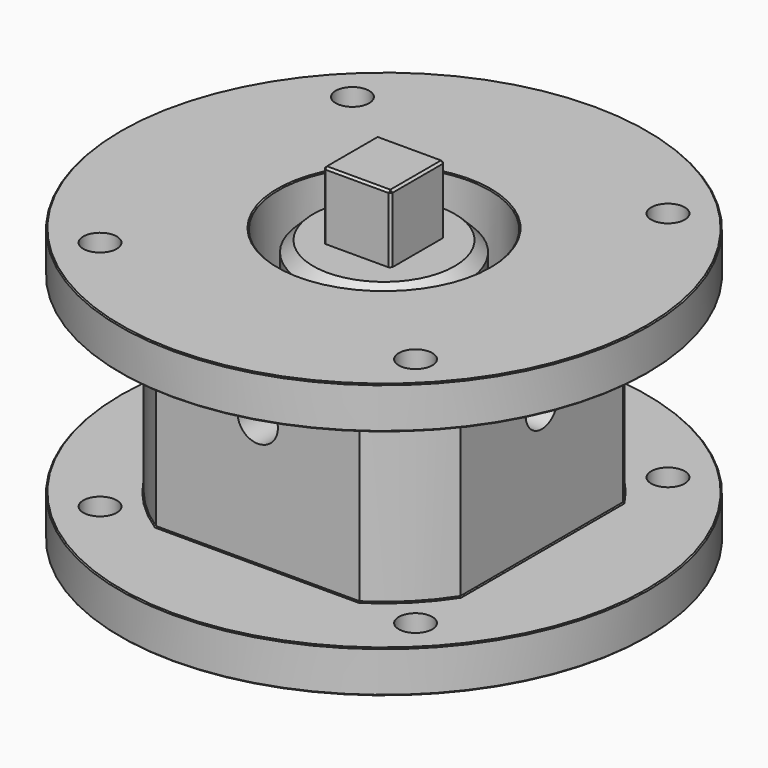
from build123d import *

# Parameters (mm, degrees)
F0_R      = 125
F0_R_2    = 50
F1_DEPTH  = 20
F2_DEPTH  = 45
F7_R      = 38.4930993585
F8_DEPTH  = 125
F9_W      = 32
F9_H      = 32
F10_DEPTH = 32
F11_W     = 32
F11_H     = 32
F12_DEPTH = 32
F13_SIZE  = 1
F14_SIZE  = 0.5
F15_D     = 15.875
F16_D     = 19.05
F16_2_D   = 19.05
F17_D     = 19.05
F17_DEPTH = 30
F17_TIP   = 5.7231973962
F19_D     = 19.05
F19_DEPTH = 30
F19_TIP   = 5.7231973962
F20_SIZE  = 5


# Not quite as in the source:
# - a length typed as a fraction of an inch, garbled in the dataset ("3 / 203.2 mm" for 3/8 in), is restored


with BuildPart() as f1:
    # F0 (on Top) → F1 (new body)
    with BuildSketch(Plane.XY):
        Circle(F0_R)
        with BuildLine():
            Line((-48.1726635133, -74.7033618391), (-74.7033618391, -74.7033618391))
            Line((-74.7033618391, -74.7033618391), (-74.7033618391, -48.1726635133))
            ThreePointArc((-74.7033618391, -48.1726635133), (-88.8886819568, 0), (-74.7033618391, 48.1726635133))
            Line((-74.7033618391, 48.1726635133), (-74.7033618391, 74.7033618391))
            Line((-74.7033618391, 74.7033618391), (-48.1726635133, 74.7033618391))
            ThreePointArc((-48.1726635133, 74.7033618391), (0, 88.8886819568), (48.1726635133, 74.7033618391))
            Line((48.1726635133, 74.7033618391), (74.7033618391, 74.7033618391))
            Line((74.7033618391, 74.7033618391), (74.7033618391, 48.1726635133))
            ThreePointArc((74.7033618391, 48.1726635133), (85.2686377036, 25.1089068699), (88.8886819568, 0))
            ThreePointArc((88.8886819568, 0), (85.2686377036, -25.1089068699), (74.7033618391, -48.1726635133))
            Line((74.7033618391, -48.1726635133), (74.7033618391, -74.7033618391))
            Line((74.7033618391, -74.7033618391), (48.1726635133, -74.7033618391))
            ThreePointArc((48.1726635133, -74.7033618391), (0, -88.8886819568), (-48.1726635133, -74.7033618391))
        make_face(mode=Mode.SUBTRACT)
        with BuildLine():
            Line((-74.7033618391, 48.1726635133), (-74.7033618391, -48.1726635133))
            ThreePointArc((-74.7033618391, -48.1726635133), (-62.8537897824, -62.8537897824), (-48.1726635133, -74.7033618391))
            Line((-48.1726635133, -74.7033618391), (48.1726635133, -74.7033618391))
            ThreePointArc((48.1726635133, -74.7033618391), (62.8537897824, -62.8537897824), (74.7033618391, -48.1726635133))
            Line((74.7033618391, -48.1726635133), (74.7033618391, 48.1726635133))
            ThreePointArc((74.7033618391, 48.1726635133), (62.8537897824, 62.8537897824), (48.1726635133, 74.7033618391))
            Line((48.1726635133, 74.7033618391), (-48.1726635133, 74.7033618391))
            ThreePointArc((-48.1726635133, 74.7033618391), (-62.8537897824, 62.8537897824), (-74.7033618391, 48.1726635133))
        make_face()
        Circle(F0_R_2, mode=Mode.SUBTRACT)
        with BuildLine():
            Line((48.1726635133, -74.7033618391), (-48.1726635133, -74.7033618391))
            ThreePointArc((-48.1726635133, -74.7033618391), (0, -88.8886819568), (48.1726635133, -74.7033618391))
        make_face()
        with BuildLine():
            ThreePointArc((-74.7033618391, 48.1726635133), (-88.8886819568, 0), (-74.7033618391, -48.1726635133))
            Line((-74.7033618391, -48.1726635133), (-74.7033618391, 48.1726635133))
        make_face()
        with BuildLine():
            ThreePointArc((48.1726635133, 74.7033618391), (0, 88.8886819568), (-48.1726635133, 74.7033618391))
            Line((-48.1726635133, 74.7033618391), (48.1726635133, 74.7033618391))
        make_face()
        with BuildLine():
            Line((74.7033618391, 48.1726635133), (74.7033618391, -48.1726635133))
            ThreePointArc((74.7033618391, -48.1726635133), (85.2686377036, -25.1089068699), (88.8886819568, 0))
            ThreePointArc((88.8886819568, 0), (85.2686377036, 25.1089068699), (74.7033618391, 48.1726635133))
        make_face()
        with BuildLine():
            Line((-74.7033618391, 74.7033618391), (-74.7033618391, 48.1726635133))
            ThreePointArc((-74.7033618391, 48.1726635133), (-62.8537897824, 62.8537897824), (-48.1726635133, 74.7033618391))
            Line((-48.1726635133, 74.7033618391), (-74.7033618391, 74.7033618391))
        make_face()
        with BuildLine():
            Line((-74.7033618391, -48.1726635133), (-74.7033618391, -74.7033618391))
            Line((-74.7033618391, -74.7033618391), (-48.1726635133, -74.7033618391))
            ThreePointArc((-48.1726635133, -74.7033618391), (-62.8537897824, -62.8537897824), (-74.7033618391, -48.1726635133))
        make_face()
        with BuildLine():
            ThreePointArc((74.7033618391, -48.1726635133), (62.8537897824, -62.8537897824), (48.1726635133, -74.7033618391))
            Line((48.1726635133, -74.7033618391), (74.7033618391, -74.7033618391))
            Line((74.7033618391, -74.7033618391), (74.7033618391, -48.1726635133))
        make_face()
        with BuildLine():
            Line((74.7033618391, 74.7033618391), (48.1726635133, 74.7033618391))
            ThreePointArc((48.1726635133, 74.7033618391), (62.8537897824, 62.8537897824), (74.7033618391, 48.1726635133))
            Line((74.7033618391, 48.1726635133), (74.7033618391, 74.7033618391))
        make_face()
    extrude(amount=-F1_DEPTH)

    # F0 (on Top) → F2 (join)
    with BuildSketch(Plane.XY):
        with BuildLine():
            Line((-74.7033618391, 48.1726635133), (-74.7033618391, -48.1726635133))
            ThreePointArc((-74.7033618391, -48.1726635133), (-62.8537897824, -62.8537897824), (-48.1726635133, -74.7033618391))
            Line((-48.1726635133, -74.7033618391), (48.1726635133, -74.7033618391))
            ThreePointArc((48.1726635133, -74.7033618391), (62.8537897824, -62.8537897824), (74.7033618391, -48.1726635133))
            Line((74.7033618391, -48.1726635133), (74.7033618391, 48.1726635133))
            ThreePointArc((74.7033618391, 48.1726635133), (62.8537897824, 62.8537897824), (48.1726635133, 74.7033618391))
            Line((48.1726635133, 74.7033618391), (-48.1726635133, 74.7033618391))
            ThreePointArc((-48.1726635133, 74.7033618391), (-62.8537897824, 62.8537897824), (-74.7033618391, 48.1726635133))
        make_face()
        Circle(F0_R_2, mode=Mode.SUBTRACT)
    extrude(amount=F2_DEPTH)

    # F3: F1 across face


with BuildPart() as f1_1:
    add(f1.part)
    add(f1.part.mirror(Plane.XY.offset(45)))

    # F14
    f14_edges = [f1_1.edges().sort_by_distance(p)[0] for p in [
        (-125, 0, 110),
        (-50, 0, 110),
        (-125, 0, 90),
        (-62.85379, 62.85379, 90),
        (-74.703362, 0, 90),
        (-62.85379, -62.85379, 90),
        (0, -74.703362, 90),
        (62.85379, -62.85379, 90),
        (74.703362, 0, 90),
        (62.85379, 62.85379, 90),
        (0, 74.703362, 90),
        (-125, 0, -20),
        (-50, 0, -20),
        (-125, 0, 0),
        (-62.85379, 62.85379, 0),
        (-74.703362, 0, 0),
        (-62.85379, -62.85379, 0),
        (0, -74.703362, 0),
        (62.85379, -62.85379, 0),
        (74.703362, 0, 0),
        (62.85379, 62.85379, 0),
        (0, 74.703362, 0),
    ]]
    chamfer(f14_edges, length=F14_SIZE)

    # F15 (through all)
    with Locations(Plane.XY.offset(110)):
        with Locations((74.7033618391, -74.7033618391), (74.7033618391, 74.7033618391), (-74.7033618391, 74.7033618391), (-74.7033618391, -74.7033618391)):
            Hole(F15_D / 2)

    # F16 (through all)
    with Locations(Plane.XZ.offset(74.7033618391)):
        with Locations((0, 60)):
            Hole(F16_D / 2)

    # F17
    with Locations(Plane.YZ.offset(74.7033618391)):
        with Locations((0, 60)):
            Hole(F17_D / 2, depth=F17_DEPTH)
            with Locations((0, 0, -(F17_DEPTH + F17_TIP / 2))):  # 118° drill point
                Cone(0, F17_D / 2, F17_TIP, mode=Mode.SUBTRACT)

    # F19
    with Locations(Plane(origin=(-74.7033618391, 0, 0), x_dir=(0, -1, 0), z_dir=(-1, 0, 0))):
        with Locations((0, 59.5)):
            Hole(F19_D / 2, depth=F19_DEPTH)
            with Locations((0, 0, -(F19_DEPTH + F19_TIP / 2))):  # 118° drill point
                Cone(0, F19_D / 2, F19_TIP, mode=Mode.SUBTRACT)


with BuildPart() as f8:
    # F7 (on face) → F8 (new body)
    with BuildSketch(Plane(origin=(0, 0, -20), x_dir=(1, 0, 0), z_dir=(0, 0, -1))):
        Circle(F7_R)
    extrude(amount=-F8_DEPTH)

    # F9 (on face) → F10 (join)
    with BuildSketch(Plane.XY.offset(105)):
        Rectangle(F9_W, F9_H)
    extrude(amount=F10_DEPTH)

    # F11 (on face) → F12 (cut)
    with BuildSketch(Plane(origin=(0, 0, -20), x_dir=(1, 0, 0), z_dir=(0, 0, -1))):
        Rectangle(F11_W, F11_H)
    extrude(amount=-F12_DEPTH, mode=Mode.SUBTRACT)

    # F13
    f13_edges = [f8.edges().sort_by_distance(p)[0] for p in [
        (-16, 16, 121),
        (-16, -16, 121),
        (16, -16, 121),
        (-16, 0, 137),
        (0, -16, 137),
        (16, 0, 137),
        (0, 16, 137),
        (16, 16, 121),
    ]]
    chamfer(f13_edges, length=F13_SIZE)

    # F16#2 (through all)
    with Locations(Plane.XZ.offset(74.7033618391)):
        with Locations((0, 60)):
            Hole(F16_2_D / 2)

    # F20
    f20_edges = [f8.edges().sort_by_distance(p)[0] for p in [
        (-38.493099, 0, 105),
    ]]
    chamfer(f20_edges, length=F20_SIZE)


solid = Compound([f1_1.part, f8.part])
